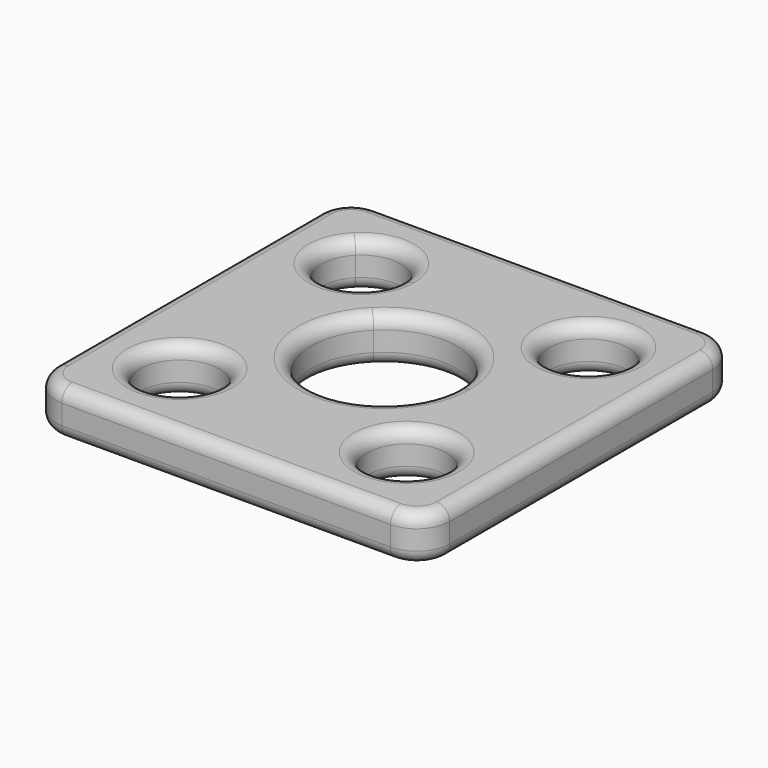
from build123d import *

# Parameters (mm, degrees)
F0_W         = 60
F0_H         = 60
F0_R         = 6
F1_DEPTH     = 7
F2_R         = 2
F3_T1_DEPTH  = 7
F3_T4_ANGLE  = 90
F3_T6_ANGLE  = 90
F3_T8_ANGLE  = 90
F3_T10_ANGLE = 90
F3_T12_ANGLE = 90
F3_T14_ANGLE = 90
F3_T16_ANGLE = 90
F3_T18_ANGLE = 90


# Not quite as in the source:
# - a fillet or chamfer that OpenCascade refuses, or shapes differently, is made with other operations: its cross-section is extruded or revolved along the edge and cut away or added


with BuildPart() as f1:
    # F0 (on Top) → F1 (new body)
    with BuildSketch(Plane.XY):
        Rectangle(F0_W, F0_H)
        with Locations((-17.2720779386, -17.2720779386)):
            Circle(F0_R, mode=Mode.SUBTRACT)
        with Locations((17.2720779386, -17.2720779386)):
            Circle(F0_R, mode=Mode.SUBTRACT)
        with BuildLine():
            ThreePointArc((-13.0294372515, 13.0294372515), (-21.5147186258, 13.0294372515), (-21.5147186258, 21.5147186258))
            ThreePointArc((-21.5147186258, 21.5147186258), (-14.9759773445, 22.8153551337), (-11.2720779386, 17.2720779386))
            ThreePointArc((-11.2720779386, 17.2720779386), (-11.7288007436, 14.9759773445), (-13.0294372515, 13.0294372515))
        make_face(mode=Mode.SUBTRACT)
        with BuildLine():
            ThreePointArc((11.05, 0), (-4.2286519276, -10.2088688342), (-7.8135299321, 7.8135299321))
            ThreePointArc((-7.8135299321, 7.8135299321), (4.2286519276, 10.2088688342), (11.05, 0))
        make_face(mode=Mode.SUBTRACT)
        with Locations((17.2720779386, 17.2720779386)):
            Circle(F0_R, mode=Mode.SUBTRACT)
    extrude(amount=F1_DEPTH)

    # F2
    f2_edges = [f1.edges().sort_by_distance(p)[0] for p in [
        (30, 0, 7),
        (0, 30, 7),
        (-30, 0, 7),
        (0, -30, 7),
        (-23.272078, -17.272078, 7),
        (11.272078, -17.272078, 7),
        (-23.272078, 17.272078, 7),
        (7.81353, -7.81353, 7),
        (11.272078, 17.272078, 7),
        (30, 0, 0),
        (0, 30, 0),
        (-30, 0, 0),
        (0, -30, 0),
        (-23.272078, -17.272078, 0),
        (11.272078, -17.272078, 0),
        (-23.272078, 17.272078, 0),
        (7.81353, -7.81353, 0),
        (11.272078, 17.272078, 0),
    ]]
    fillet(f2_edges, radius=F2_R)

    # F3: fillet of radius 5 on 4 edges, made by hand

    # F3_s2 → F3_t1 (cut)
    with BuildSketch(Plane.XY):
        with BuildLine():
            ThreePointArc((-25, -30), (-28.5355339059, -28.5355339059), (-30, -25))
            Line((-30, -25), (-30, -30))
            Line((-30, -30), (-25, -30))
        make_face()
        with BuildLine():
            ThreePointArc((-25, 30), (-28.5355339059, 28.5355339059), (-30, 25))
            Line((-30, 25), (-30, 30))
            Line((-30, 30), (-25, 30))
        make_face()
        with BuildLine():
            ThreePointArc((30, 25), (28.5355339059, 28.5355339059), (25, 30))
            Line((25, 30), (30, 30))
            Line((30, 30), (30, 25))
        make_face()
        with BuildLine():
            ThreePointArc((30, -25), (28.5355339059, -28.5355339059), (25, -30))
            Line((25, -30), (30, -30))
            Line((30, -30), (30, -25))
        make_face()
    extrude(amount=F3_T1_DEPTH, mode=Mode.SUBTRACT)

    # F3_s3 → F3_t4 (revolve, cut)
    with BuildSketch(Plane.XZ.offset(25)):
        with BuildLine():
            ThreePointArc((28, 0), (29.4142135624, 0.5857864376), (30, 2))
            Line((30, 2), (30, 0))
            Line((30, 0), (28, 0))
        make_face()
    revolve(axis=Axis((25, -25, 0), (0, 0, -1)), revolution_arc=F3_T4_ANGLE, mode=Mode.SUBTRACT)

    # F3_s5 → F3_t6 (revolve, cut)
    with BuildSketch(Plane.YZ.offset(25)):
        with BuildLine():
            ThreePointArc((-28, 7), (-29.4142135624, 6.4142135624), (-30, 5))
            Line((-30, 5), (-30, 7))
            Line((-30, 7), (-28, 7))
        make_face()
    revolve(axis=Axis((25, -25, 7), (0, 0, 1)), revolution_arc=F3_T6_ANGLE, mode=Mode.SUBTRACT)

    # F3_s7 → F3_t8 (revolve, cut)
    with BuildSketch(Plane.YZ.offset(25)):
        with BuildLine():
            ThreePointArc((28, 0), (29.4142135624, 0.5857864376), (30, 2))
            Line((30, 2), (30, 0))
            Line((30, 0), (28, 0))
        make_face()
    revolve(axis=Axis((25, 25, 0), (0, 0, -1)), revolution_arc=F3_T8_ANGLE, mode=Mode.SUBTRACT)

    # F3_s9 → F3_t10 (revolve, cut)
    with BuildSketch(Plane.XZ.offset(-25)):
        with BuildLine():
            ThreePointArc((28, 7), (29.4142135624, 6.4142135624), (30, 5))
            Line((30, 5), (30, 7))
            Line((30, 7), (28, 7))
        make_face()
    revolve(axis=Axis((25, 25, 7), (0, 0, 1)), revolution_arc=F3_T10_ANGLE, mode=Mode.SUBTRACT)

    # F3_s11 → F3_t12 (revolve, cut)
    with BuildSketch(Plane.XZ.offset(-25)):
        with BuildLine():
            ThreePointArc((-28, 0), (-29.4142135624, 0.5857864376), (-30, 2))
            Line((-30, 2), (-30, 0))
            Line((-30, 0), (-28, 0))
        make_face()
    revolve(axis=Axis((-25, 25, 0), (0, 0, -1)), revolution_arc=F3_T12_ANGLE, mode=Mode.SUBTRACT)

    # F3_s13 → F3_t14 (revolve, cut)
    with BuildSketch(Plane.YZ.offset(-25)):
        with BuildLine():
            ThreePointArc((28, 7), (29.4142135624, 6.4142135624), (30, 5))
            Line((30, 5), (30, 7))
            Line((30, 7), (28, 7))
        make_face()
    revolve(axis=Axis((-25, 25, 7), (0, 0, 1)), revolution_arc=F3_T14_ANGLE, mode=Mode.SUBTRACT)

    # F3_s15 → F3_t16 (revolve, cut)
    with BuildSketch(Plane.YZ.offset(-25)):
        with BuildLine():
            ThreePointArc((-28, 0), (-29.4142135624, 0.5857864376), (-30, 2))
            Line((-30, 2), (-30, 0))
            Line((-30, 0), (-28, 0))
        make_face()
    revolve(axis=Axis((-25, -25, 0), (0, 0, -1)), revolution_arc=F3_T16_ANGLE, mode=Mode.SUBTRACT)

    # F3_s17 → F3_t18 (revolve, cut)
    with BuildSketch(Plane.XZ.offset(25)):
        with BuildLine():
            ThreePointArc((-28, 7), (-29.4142135624, 6.4142135624), (-30, 5))
            Line((-30, 5), (-30, 7))
            Line((-30, 7), (-28, 7))
        make_face()
    revolve(axis=Axis((-25, -25, 7), (0, 0, 1)), revolution_arc=F3_T18_ANGLE, mode=Mode.SUBTRACT)


solid = f1.part
